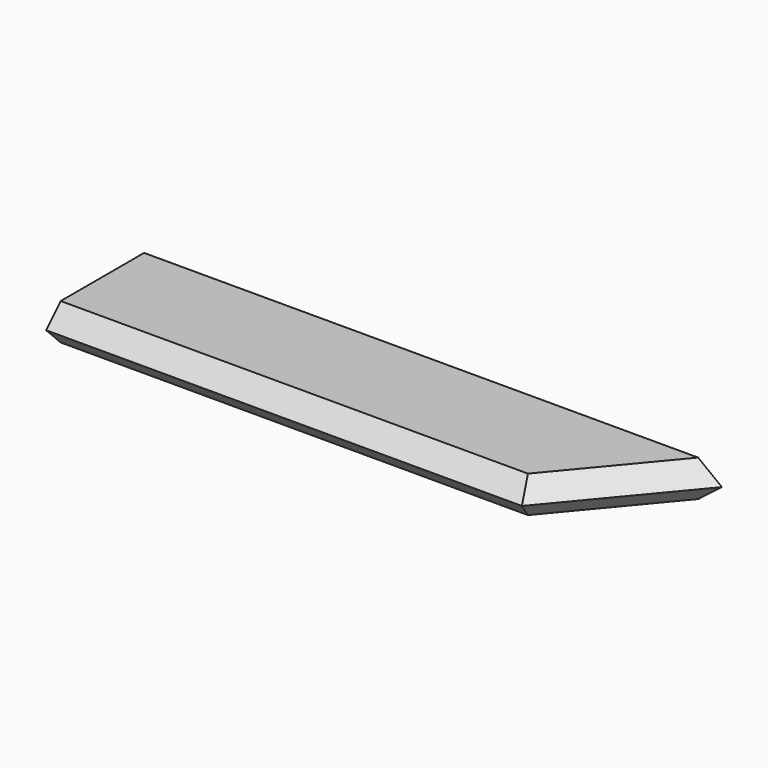
from build123d import *

# Parameters (mm, degrees)
F1_DEPTH = 3.556
F2_SIZE  = 1.77799


# Not quite as in the source:
# - a fillet or chamfer is up to 0.001 mm smaller than in the source, because OpenCascade refuses the exact size


with BuildPart() as f1:
    # F0 (on Top) → F1 (new body)
    with BuildSketch(Plane.XY):
        Polygon((-43.0519394577, 11.9240293279), (-43.0519394577, 0), (3.2667792402, 0), (13.2010905072, 11.9240293279), align=None)
    extrude(amount=F1_DEPTH)

    # F2 (size 1.778 in the source; OpenCascade refuses exactly that, so slightly less here)
    f2_edges = [f1.edges().sort_by_distance(p)[0] for p in [
        (8.233935, 5.962015, 0),
        (8.233935, 5.962015, 3.556),
        (-19.89258, 0, 0),
        (-19.89258, 0, 3.556),
    ]]
    chamfer(f2_edges, length=F2_SIZE)


solid = f1.part
